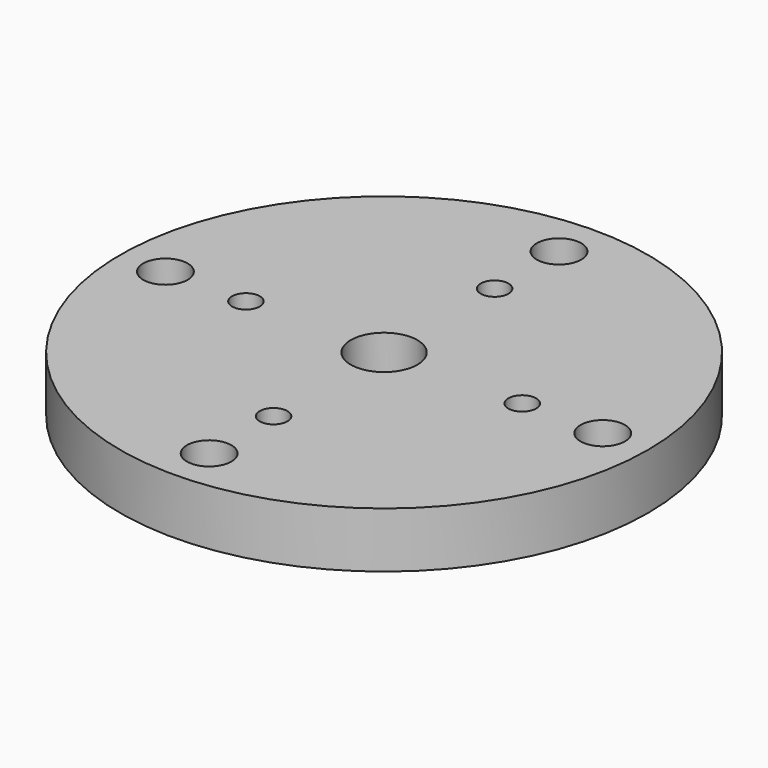
from build123d import *

# Parameters (mm, degrees)
F0_R      = 47.5
F1_DEPTH  = 45
F2_W      = 40.64
F2_H      = 40.64
F3_DEPTH  = 35
F4_R      = 6
F6_DEPTH  = 10.001
F7_W      = 7.9080420285
F7_H      = 7.9080420285
F8_DEPTH  = 35
F9_R      = 4
F10_DEPTH = 10.001
F11_DEPTH = 35
F12_R     = 2.5
F13_DEPTH = 10.001


with BuildPart() as f1:
    # F0 (on Top) → F1 (new body)
    with BuildSketch(Plane.XY):
        Circle(F0_R)
    extrude(amount=F1_DEPTH)

    # F2 (on face) → F3 (cut)
    with BuildSketch(Plane.XY.offset(45)):
        Rectangle(F2_W, F2_H)
    extrude(amount=-F3_DEPTH, mode=Mode.SUBTRACT)

    # F4 (on face) → F6 (cut, through all)
    with BuildSketch(Plane.XY.offset(10)):
        Circle(F4_R)
    extrude(amount=-F6_DEPTH, mode=Mode.SUBTRACT)

    # F7 (on face) → F8 (cut)
    with BuildSketch(Plane.XY.offset(45)):
        Polygon((37.3080420285, 37.3080420285), (37.3080420285, 29.4), (29.4, 29.4), (29.4, -29.4), (37.3080420285, -29.4), (37.3080420285, -37.3080420285), (49.4, -37.3080420285), (49.4, 37.3080420285), align=None)
        with Locations((33.3540210142, 33.3540210142)):
            Rectangle(F7_W, F7_H)
        Polygon((-29.4, 29.4), (29.4, 29.4), (29.4, 37.3080420285), (37.3080420285, 37.3080420285), (37.3080420285, 49.4), (-37.3080420285, 49.4), (-37.3080420285, 37.3080420285), (-29.4, 37.3080420285), align=None)
        Polygon((-29.4, -29.4), (-29.4, 29.4), (-37.3080420285, 29.4), (-37.3080420285, 37.3080420285), (-49.4, 37.3080420285), (-49.4, -37.3080420285), (-37.3080420285, -37.3080420285), (-37.3080420285, -29.4), align=None)
        with Locations((-33.3540210142, 33.3540210142)):
            Rectangle(F7_W, F7_H)
        Polygon((29.4, -37.3080420285), (29.4, -29.4), (-29.4, -29.4), (-29.4, -37.3080420285), (-37.3080420285, -37.3080420285), (-37.3080420285, -49.4), (37.3080420285, -49.4), (37.3080420285, -37.3080420285), align=None)
        with Locations((33.3540210142, -33.3540210142)):
            Rectangle(F7_W, F7_H)
        with Locations((-33.3540210142, -33.3540210142)):
            Rectangle(F7_W, F7_H)
    extrude(amount=-F8_DEPTH, mode=Mode.SUBTRACT)

    # F9 (on face) → F10 (cut, through all)
    with BuildSketch(Plane.XY.offset(10)):
        with Locations((0, 39.35)):
            Circle(F9_R)
        with Locations((39.35, 0)):
            Circle(F9_R)
        with Locations((0, -39.35)):
            Circle(F9_R)
        with Locations((-39.35, 0)):
            Circle(F9_R)
    extrude(amount=-F10_DEPTH, mode=Mode.SUBTRACT)

    # F11 (cut): a face of the model
    f11_faces = [f1.faces().sort_by_distance(p)[0] for p in [
        (0, -28.5684424253, 45),
    ]]
    extrude(f11_faces, amount=-F11_DEPTH, mode=Mode.SUBTRACT)

    # F12 (on face) → F13 (cut, through all)
    with BuildSketch(Plane(origin=(0, 0, 0), x_dir=(1, 0, 0), z_dir=(0, 0, -1))):
        with Locations((0, 24.86)):
            Circle(F12_R)
        with Locations((24.86, 0)):
            Circle(F12_R)
        with Locations((0, -24.86)):
            Circle(F12_R)
        with Locations((-24.86, 0)):
            Circle(F12_R)
    extrude(amount=-F13_DEPTH, mode=Mode.SUBTRACT)


solid = f1.part
